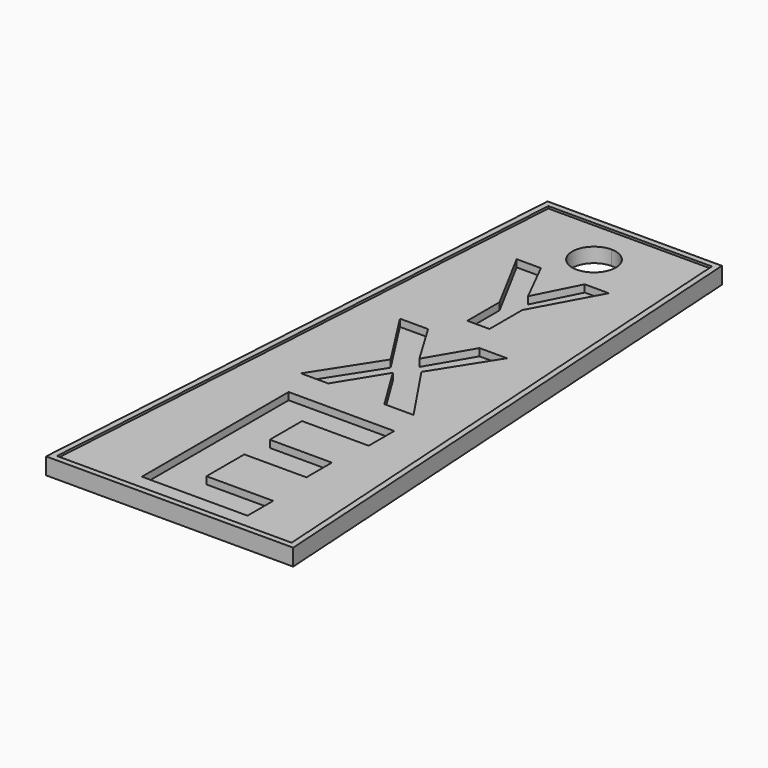
from build123d import *

# Parameters (mm, degrees)
F1_DEPTH       = 2
F2_TEXT_SIZE   = 35.349351008
F2_TEXT_SIZE_2 = 23.2280102477
F2_TEXT_SIZE_3 = 20.3220684963
F3_DEPTH       = 1
F5_DEPTH       = 0.3


# Not quite as in the source:
# - Text() gives the source's letters only with a copy of the font that has no kerning and outlines rounded to 1/6400 em; it was checked with that copy


with BuildPart() as f1:
    # F0 (on Top) → F1 (new body)
    with BuildSketch(Plane.XY):
        with BuildLine():
            Line((0, 40.9355648028), (0, 44.9355648028))
            Line((0, 44.9355648028), (-12, 44.9355648028))
            Line((-12, 44.9355648028), (-17, -35.0644351972))
            Line((-17, -35.0644351972), (0, -35.0644351972))
            Line((0, -35.0644351972), (0, 0))
            Line((0, 0), (0, 34.9355648028))
            ThreePointArc((0, 34.9355648028), (-3, 37.9355648028), (0, 40.9355648028))
        make_face()
        with BuildLine():
            Line((12, 44.9355648028), (0, 44.9355648028))
            Line((0, 44.9355648028), (0, 40.9355648028))
            ThreePointArc((0, 40.9355648028), (2.1213203436, 40.0568851463), (3, 37.9355648028))
            ThreePointArc((3, 37.9355648028), (2.1213203436, 35.8142444592), (0, 34.9355648028))
            Line((0, 34.9355648028), (0, 0))
            Line((0, 0), (0, -35.0644351972))
            Line((0, -35.0644351972), (17, -35.0644351972))
            Line((17, -35.0644351972), (12, 44.9355648028))
        make_face()
    extrude(amount=F1_DEPTH)

    # F2 (on face) → F3 (cut)
    with BuildSketch(Plane.XY.offset(2)):
        with Locations((-9.5454674983, -31.8720246186)):
            Text('E', F2_TEXT_SIZE, font='Open Sans', font_style=FontStyle.BOLD, text_align=(TextAlign.LEFT, TextAlign.BOTTOM))
        with Locations((-8.0454674983, -2.4204918928)):
            Text('X', F2_TEXT_SIZE_2, font='Open Sans', font_style=FontStyle.BOLD, text_align=(TextAlign.LEFT, TextAlign.BOTTOM))
        with Locations((-6.5454674983, 18.3036754855)):
            Text('Y', F2_TEXT_SIZE_3, font='Open Sans', font_style=FontStyle.BOLD, text_align=(TextAlign.LEFT, TextAlign.BOTTOM))
    extrude(amount=-F3_DEPTH, mode=Mode.SUBTRACT)

    # F4 (on face) → F5 (join)
    with BuildSketch(Plane.XY.offset(2)):
        Polygon((12, 44.9355648028), (-12, 44.9355648028), (-17, -35.0644351972), (17, -35.0644351972), align=None)
        Polygon((-11.2484390229, 44.1355648028), (11.2484390229, 44.1355648028), (16.1484390229, -34.2644351972), (-16.1484390229, -34.2644351972), align=None, mode=Mode.SUBTRACT)
    extrude(amount=F5_DEPTH)


solid = f1.part
